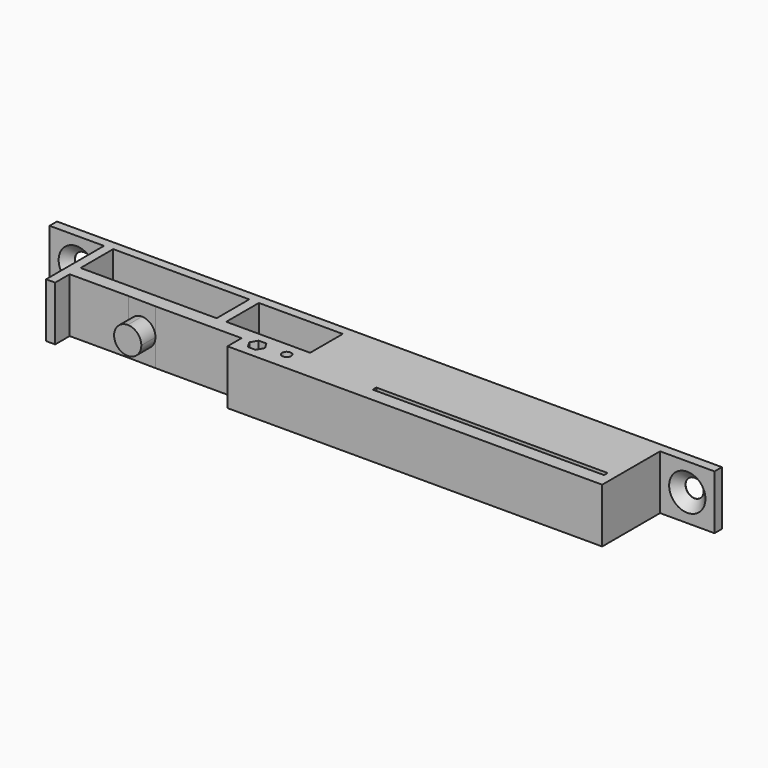
from build123d import *

# Parameters (mm, degrees)
F7_DEPTH  = 12
F3_W      = 18.5
F3_H      = 9
F5_R      = 1
F2_W      = 30
F2_H      = 9
F0_W      = 51
F0_H      = 1
F8_DEPTH  = 12
F9_DEPTH  = 9
F10_DEPTH = 3
F11_R     = 2.99999
F13_R     = 2
F12_R     = 2
F14_DEPTH = 23.9
F15_SIZE  = 2
F1_W      = 13
F1_H      = 13
F16_DEPTH = 10


# Not quite as in the source:
# - a fillet or chamfer is up to 0.001 mm smaller than in the source, because OpenCascade refuses the exact size


with BuildPart() as f7:
    # F6 (on Top) → F7 (new body)
    with BuildSketch(Plane.XY):
        Polygon((58.3547055721, 23.1172949925), (-78.9411039278, 23.1172949925), (-78.9411039278, 21.0728161037), (-66.9411039278, 21.0728161037), (-66.9411039278, 5.1172949925), (-64.9411039278, 5.1172949925), (-64.9411039278, 9.1172949925), (-51.9411039278, 9.1172949925), (-45.9411039278, 9.0077459167), (-26.9411039278, 9.0077459167), (-26.9411039278, 5.1172949925), (55.6804920286, 5.1172949925), (55.6804920286, 21.0728161037), (67.6804920286, 21.0728161037), (67.6804920286, 23.1172949925), align=None)
    extrude(amount=F7_DEPTH)

    # F4 (on Top) + F3 (on Top) + F5 (on Top) + F2 (on Top) + F0 (on Top) → F8 (cut)
    with BuildSketch(Plane.XY):
        Polygon((-22.3430277164, 7.1172949925), (-21.4770023127, 8.6172949925), (-22.3430277164, 10.1172949925), (-24.075078524, 10.1172949925), (-24.9411039278, 8.6172949925), (-24.075078524, 7.1172949925), align=None)
    with BuildSketch(Plane.XY):
        with Locations((-23.5695079714, 16.6172949925)):
            Rectangle(F3_W, F3_H)
    with BuildSketch(Plane.XY):
        with Locations((-17.0899687546, 9.1172949925)):
            Circle(F5_R)
    with BuildSketch(Plane.XY):
        with Locations((-49.9411039278, 16.6172949925)):
            Rectangle(F2_W, F2_H)
    with BuildSketch(Plane.XY):
        with Locations((28.1804920286, 8.6172949925)):
            Rectangle(F0_W, F0_H)
    extrude(amount=F8_DEPTH, mode=Mode.SUBTRACT)

    # F6 (on Top) → F9 (join)
    with BuildSketch(Plane.XY):
        Polygon((-51.9411039278, 9.1172949925), (-51.9411039278, 5.1172949925), (-45.9411039278, 5.1172949925), (-45.9411039278, 9.0077459167), align=None)
    extrude(amount=F9_DEPTH)

    # F6 (on Top) → F10 (cut)
    with BuildSketch(Plane.XY):
        Polygon((-51.9411039278, 9.1172949925), (-51.9411039278, 5.1172949925), (-45.9411039278, 5.1172949925), (-45.9411039278, 9.0077459167), align=None)
    extrude(amount=F10_DEPTH, mode=Mode.SUBTRACT)

    # F11 (radius 3 in the source; OpenCascade refuses exactly that, so slightly less here)
    f11_edges = [f7.edges().sort_by_distance(p)[0] for p in [
        (-51.941104, 7.117295, 9),
        (-45.941104, 7.06252, 9),
        (-51.941104, 7.117295, 3),
        (-45.941104, 7.06252, 3),
    ]]
    fillet(f11_edges, radius=F11_R)

    # F13 (on Front) + F12 (on Front) → F14 (cut)
    with BuildSketch(Plane.XZ):
        with Locations((-72.9411039278, 6)):
            Circle(F13_R)
    with BuildSketch(Plane.XZ):
        with Locations((61.6804920286, 6)):
            Circle(F12_R)
    extrude(amount=-F14_DEPTH, mode=Mode.SUBTRACT)

    # F15
    f15_edges = [f7.edges().sort_by_distance(p)[0] for p in [
        (-74.941104, 21.072816, 6),
        (59.680492, 21.072816, 6),
    ]]
    chamfer(f15_edges, length=F15_SIZE)

    # F1 (on Top) → F16 (cut)
    with BuildSketch(Plane.XY):
        with Locations((-5.8195079714, 14.6172949925)):
            Rectangle(F1_W, F1_H)
    extrude(amount=F16_DEPTH, mode=Mode.SUBTRACT)


solid = f7.part
